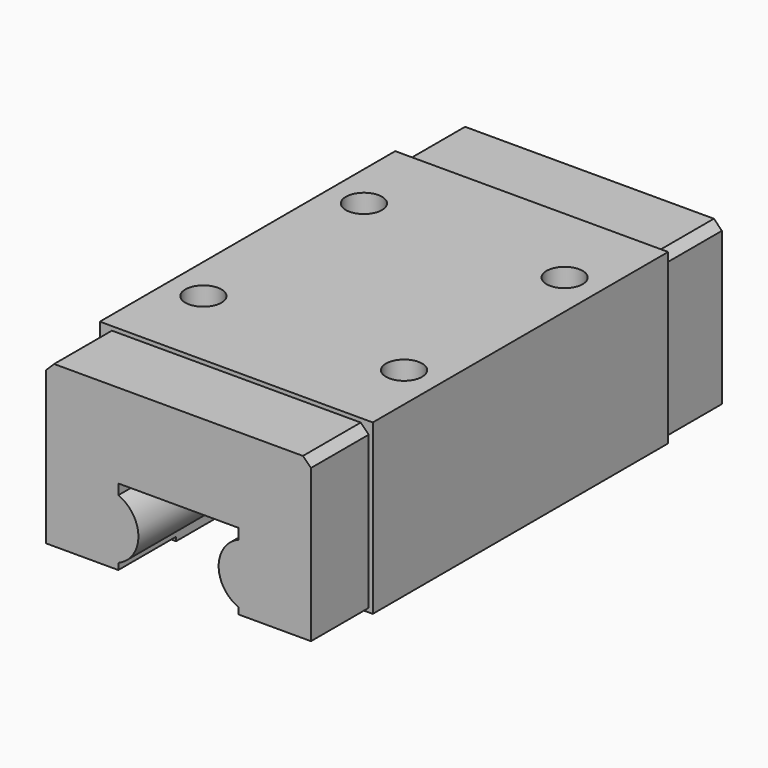
from build123d import *

# Parameters (mm, degrees)
F1_DEPTH = 32
F2_W     = 34
F2_H     = 21
F3_DEPTH = 9
F5_D     = 4.5
F5_DEPTH = 10.4
F5_TIP   = 1.3519363928


# Not quite as in the source:
# - a pattern or mirror of a feature is missing from the dataset's text; its kind, count and spacing are read off the source's solid


with BuildPart() as f1:
    # F0 (on Front) → F1 (new body, symmetric)
    with BuildSketch(Plane.XZ):
        with BuildLine():
            Line((-17, 21), (-17, 0))
            Line((-17, 0), (-7.5, 0))
            Line((-7.5, 0), (-7.5, 1.2919007565))
            ThreePointArc((-7.5, 1.2919007565), (-5, 5), (-7.5, 8.7080992435))
            Line((-7.5, 8.7080992435), (-7.5, 10))
            Line((-7.5, 10), (7.5, 10))
            Line((7.5, 10), (7.5, 8.7080992435))
            ThreePointArc((7.5, 8.7080992435), (5, 5), (7.5, 1.2919007565))
            Line((7.5, 1.2919007565), (7.5, 0))
            Line((7.5, 0), (17, 0))
            Line((17, 0), (17, 21))
            Line((17, 21), (-17, 21))
        make_face()
    extrude(amount=F1_DEPTH, both=True)

    # F2 (on face) → F3 (cut)
    with BuildSketch(Plane.XZ.offset(32)):
        with Locations((0, 10.5)):
            Rectangle(F2_W, F2_H)
        Polygon((-16.5, 19.5), (-15.5, 20.5), (15.5, 20.5), (16.5, 19.5), (16.5, 0.5), (-16.5, 0.5), align=None, mode=Mode.SUBTRACT)
    f3 = extrude(amount=-F3_DEPTH, mode=Mode.SUBTRACT)

    # F3_copies: F3 across plane
    add(f3.mirror(Plane.ZX), mode=Mode.SUBTRACT)

    # F5
    with Locations(Plane.XY.offset(21)):
        with Locations((-12.5, 12.5), (12.5, 12.5), (12.5, -12.5), (-12.5, -12.5)):
            Hole(F5_D / 2, depth=F5_DEPTH)
            with Locations((0, 0, -(F5_DEPTH + F5_TIP / 2))):  # 118° drill point
                Cone(0, F5_D / 2, F5_TIP, mode=Mode.SUBTRACT)


solid = f1.part
